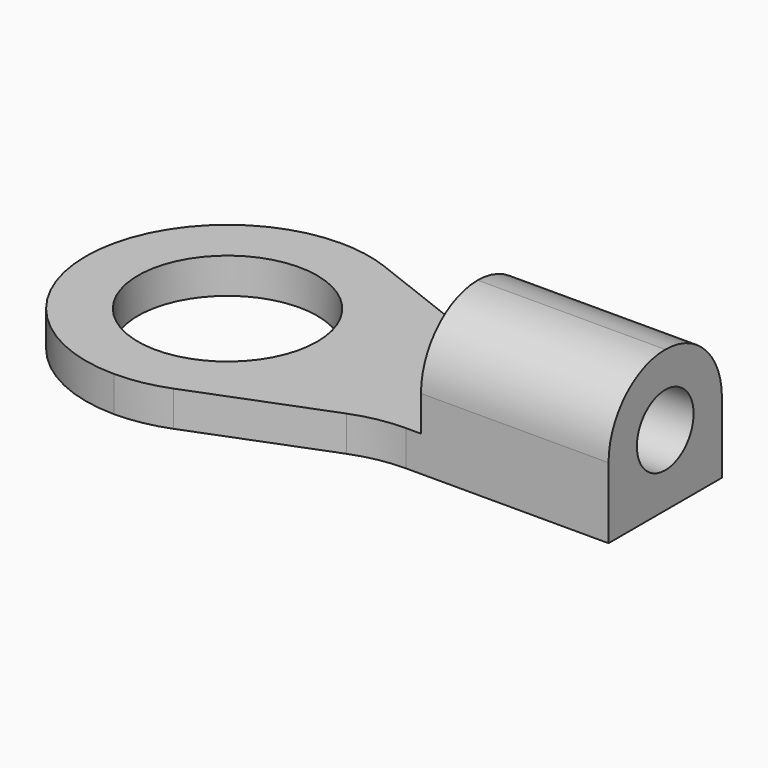
from build123d import *

# Parameters (mm, degrees)
F0_R     = 2.15
F1_DEPTH = 0.85
F2_W     = 4.5
F2_H     = 3.4
F3_DEPTH = 2.55
F4_R     = 1.69999
F5_R     = 0.85
F6_DEPTH = 25


# Not quite as in the source:
# - a fillet or chamfer is up to 0.001 mm smaller than in the source, because OpenCascade refuses the exact size


with BuildPart() as f1:
    # F0 (on Top) → F1 (new body)
    with BuildSketch(Plane.XY):
        with BuildLine():
            Line((9.0393070198, 1.7), (13.9, 1.7))
            Line((13.9, 1.7), (13.9, 5.1))
            Line((13.9, 5.1), (9.0393070198, 5.1))
            ThreePointArc((9.0393070198, 5.1), (8.4110104984, 5.1585566769), (7.8043557161, 5.332209717))
            Line((7.8043557161, 5.332209717), (4.6349513038, 6.567790283))
            ThreePointArc((4.6349513038, 6.567790283), (4.0282965214, 6.7414433231), (3.4, 6.8))
            ThreePointArc((3.4, 6.8), (0.995836944, 5.804163056), (0, 3.4))
            ThreePointArc((0, 3.4), (0.995836944, 0.995836944), (3.4, 0))
            ThreePointArc((3.4, 0), (4.0282965214, 0.0585566769), (4.6349513038, 0.232209717))
            Line((4.6349513038, 0.232209717), (7.8043557161, 1.467790283))
            ThreePointArc((7.8043557161, 1.467790283), (8.4110104984, 1.6414433231), (9.0393070198, 1.7))
        make_face()
        with Locations((3.4, 3.4)):
            Circle(F0_R, mode=Mode.SUBTRACT)
    extrude(amount=F1_DEPTH)

    # F2 (on face) → F3 (join)
    with BuildSketch(Plane.XY.offset(0.85)):
        with Locations((11.65, 3.4)):
            Rectangle(F2_W, F2_H)
    extrude(amount=F3_DEPTH)

    # F4 (radius 1.7 in the source; OpenCascade refuses exactly that, so slightly less here)
    f4_edges = [f1.edges().sort_by_distance(p)[0] for p in [
        (11.65, 5.1, 3.4),
        (11.65, 1.7, 3.4),
    ]]
    fillet(f4_edges, radius=F4_R)

    # F5 (on face) → F6 (cut)
    with BuildSketch(Plane.YZ.offset(13.9)):
        with Locations((3.4, 1.7)):
            Circle(F5_R)
    extrude(amount=-F6_DEPTH, mode=Mode.SUBTRACT)


solid = f1.part
